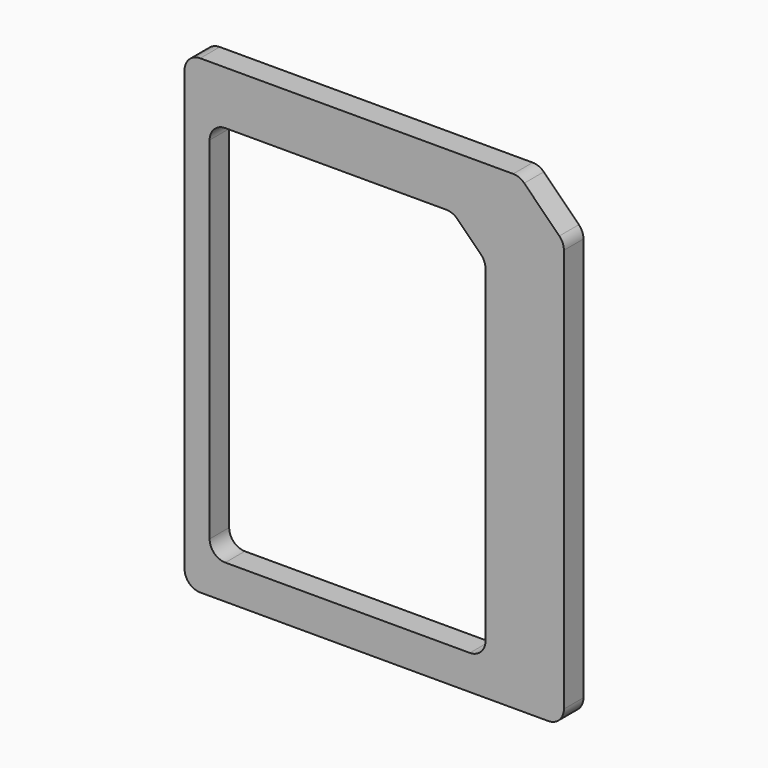
from build123d import *

# Parameters (mm, degrees)
F1_DEPTH = 0.78
F2_R     = 0.5
F4_DEPTH = 25
F5_R     = 0.5


with BuildPart() as f1:
    # F0 (on Front) → F1 (new body)
    with BuildSketch(Plane.XZ):
        Polygon((4.6385581188, 7.5), (-6.05, 7.5), (-6.05, -7.5), (6.05, -7.5), (6.05, 6.0885581188), align=None)
    extrude(amount=F1_DEPTH)

    # F2
    f2_edges = [f1.edges().sort_by_distance(p)[0] for p in [
        (-6.05, -0.39, 7.5),
        (-6.05, -0.39, -7.5),
        (6.05, -0.39, -7.5),
        (4.638558, -0.39, 7.5),
        (6.05, -0.39, 6.088558),
    ]]
    fillet(f2_edges, radius=F2_R)

    # F3 (on face) → F4 (cut)
    with BuildSketch(Plane.XZ.offset(0.78)):
        Polygon((2.5064539127, 5.8), (-5.25, 5.8), (-5.25, -6.4), (3.55, -6.4), (3.55, 4.7564539127), align=None)
    extrude(amount=-F4_DEPTH, mode=Mode.SUBTRACT)

    # F5
    f5_edges = [f1.edges().sort_by_distance(p)[0] for p in [
        (-5.25, -0.39, 5.8),
        (-5.25, -0.39, -6.4),
        (3.55, -0.39, -6.4),
        (3.55, -0.39, 4.756454),
        (2.506454, -0.39, 5.8),
    ]]
    fillet(f5_edges, radius=F5_R)


solid = f1.part
